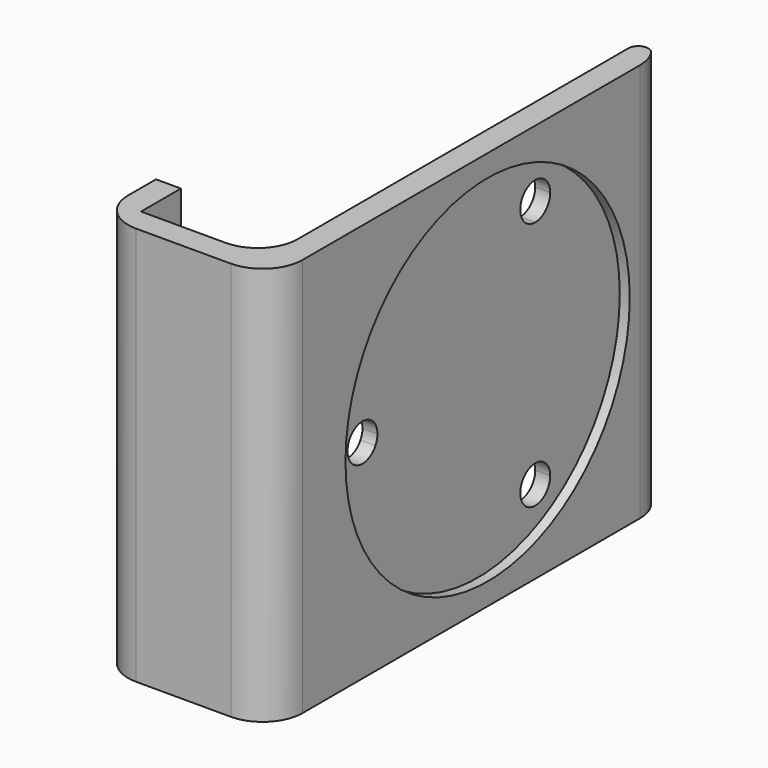
from build123d import *

# Parameters (mm, degrees)
F0_W        = 63.5
F0_H        = 50.8
F1_DEPTH    = 3.175
F2_R        = 22.621875
F3_DEPTH    = 1.27
F5_DEPTH    = 25.4
F7_DEPTH    = 50.8
F8_T1_DEPTH = 50.8
F8_T3_DEPTH = 74.3464301965
F8_T5_DEPTH = 76.2
F9_R        = 5.08
F10_R       = 1.27


# Not quite as in the source:
# - a fillet or chamfer that OpenCascade refuses, or shapes differently, is made with other operations: its cross-section is extruded or revolved along the edge and cut away or added


with BuildPart() as f1:
    # F0 (on Right) → F1 (new body)
    with BuildSketch(Plane.YZ):
        Rectangle(F0_W, F0_H)
    extrude(amount=F1_DEPTH)

    # F2 (on face) → F3 (cut)
    with BuildSketch(Plane.YZ.offset(3.175)):
        with Locations((2.778125, 0)):
            Circle(F2_R)
    extrude(amount=-F3_DEPTH, mode=Mode.SUBTRACT)

    # F4 (on face) → F5 (cut)
    with BuildSketch(Plane.YZ.offset(1.905)):
        with BuildLine():
            ThreePointArc((14.3248105234, 15.875), (11.3272476722, 18.1751108739), (9.8813375306, 14.684375))
            Line((9.8813375306, 14.684375), (11.9435605234, 15.875))
            Line((11.9435605234, 15.875), (11.9435605234, 13.49375))
            ThreePointArc((11.9435605234, 13.49375), (13.6273585461, 14.1912019773), (14.3248105234, 15.875))
        make_face()
        with BuildLine():
            Line((-15.5527460468, 0), (-13.490523054, 1.190625))
            ThreePointArc((-13.490523054, 1.190625), (-17.9339960468, 0), (-13.490523054, -1.190625))
            Line((-13.490523054, -1.190625), (-15.5527460468, 0))
        make_face()
        with BuildLine():
            ThreePointArc((-13.490523054, -1.190625), (-13.2526351729, -0.6163128512), (-13.1714960468, 0))
            Line((-13.1714960468, 0), (-15.5527460468, 0))
            Line((-15.5527460468, 0), (-13.490523054, -1.190625))
        make_face()
        with BuildLine():
            Line((-15.5527460468, 0), (-13.1714960468, 0))
            ThreePointArc((-13.1714960468, 0), (-13.2526351729, 0.6163128512), (-13.490523054, 1.190625))
            Line((-13.490523054, 1.190625), (-15.5527460468, 0))
        make_face()
        with BuildLine():
            ThreePointArc((10.7529355234, -13.8127770072), (10.2597625007, -14.1912019773), (9.8813375306, -14.684375))
            Line((9.8813375306, -14.684375), (11.9435605234, -15.875))
            Line((11.9435605234, -15.875), (10.7529355234, -13.8127770072))
        make_face()
        with BuildLine():
            Line((11.9435605234, 15.875), (10.7529355234, 13.8127770072))
            ThreePointArc((10.7529355234, 13.8127770072), (11.3272476722, 13.5748891261), (11.9435605234, 13.49375))
            Line((11.9435605234, 13.49375), (11.9435605234, 15.875))
        make_face()
        with BuildLine():
            Line((11.9435605234, 15.875), (9.8813375306, 14.684375))
            ThreePointArc((9.8813375306, 14.684375), (10.2597625007, 14.1912019773), (10.7529355234, 13.8127770072))
            Line((10.7529355234, 13.8127770072), (11.9435605234, 15.875))
        make_face()
        with BuildLine():
            Line((11.9435605234, -15.875), (9.8813375306, -14.684375))
            ThreePointArc((9.8813375306, -14.684375), (11.3272476722, -18.1751108739), (14.3248105234, -15.875))
            ThreePointArc((14.3248105234, -15.875), (13.6273585461, -14.1912019773), (11.9435605234, -13.49375))
            Line((11.9435605234, -13.49375), (11.9435605234, -15.875))
        make_face()
        with BuildLine():
            ThreePointArc((11.9435605234, -13.49375), (11.3272476722, -13.5748891261), (10.7529355234, -13.8127770072))
            Line((10.7529355234, -13.8127770072), (11.9435605234, -15.875))
            Line((11.9435605234, -15.875), (11.9435605234, -13.49375))
        make_face()
    extrude(amount=-F5_DEPTH, mode=Mode.SUBTRACT)

    # F6 (on face) → F7 (join, through all)
    with BuildSketch(Plane.XY.offset(25.4)):
        Polygon((-19.05, -31.75), (0, -31.75), (0, -28.575), (-15.875, -28.575), (-15.875, -22.225), (-19.05, -22.225), align=None)
    extrude(amount=-F7_DEPTH)

    # F8: fillet of radius 5.08 on 3 edges, made by hand

    # F8_s2 → F8_t1 (join)
    with BuildSketch(Plane.XY.offset(-25.4)):
        with BuildLine():
            ThreePointArc((-5.08, -28.575), (-1.4878975516, -27.0871024484), (0, -23.495))
            Line((0, -23.495), (0, -28.575))
            Line((0, -28.575), (-5.08, -28.575))
        make_face()
    extrude(amount=F8_T1_DEPTH)

    # F8_s4 → F8_t3 (cut)
    with BuildSketch(Plane.XY.offset(-37.1732150983)):
        with BuildLine():
            ThreePointArc((0, 31.75), (2.3071134838, 29.8805202921), (3.175, 27.0407139607))
            Line((3.175, 27.0407139607), (3.175, 31.75))
            Line((3.175, 31.75), (0, 31.75))
        make_face()
    extrude(amount=F8_T3_DEPTH, mode=Mode.SUBTRACT)

    # F8_s6 → F8_t5 (cut)
    with BuildSketch(Plane.XY.offset(-38.1)):
        with BuildLine():
            ThreePointArc((-19.05, -26.67), (-17.5621024484, -30.2621024484), (-13.97, -31.75))
            Line((-13.97, -31.75), (-19.05, -31.75))
            Line((-19.05, -31.75), (-19.05, -26.67))
        make_face()
    extrude(amount=F8_T5_DEPTH, mode=Mode.SUBTRACT)

    # F9
    f9_edges = [f1.edges().sort_by_distance(p)[0] for p in [
        (3.175, -31.75, 0),
    ]]
    fillet(f9_edges, radius=F9_R)

    # F10
    f10_edges = [f1.edges().sort_by_distance(p)[0] for p in [
        (0, 31.75, 0),
    ]]
    fillet(f10_edges, radius=F10_R)


solid = f1.part
